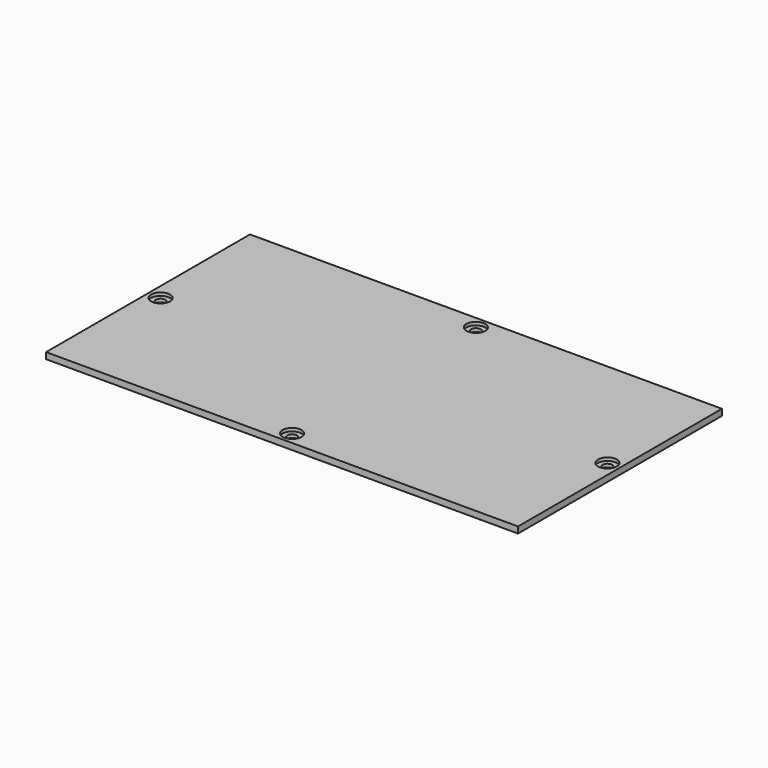
from build123d import *

# Parameters (mm, degrees)
F0_W     = 8
F0_H     = 8
F0_R     = 3
F1_DEPTH = 2
F0_R_2   = 1.5
F2_DEPTH = 1


# Not quite as in the source:
# - a feature names something its author has since deleted; it is built from what else it names


with BuildPart() as f1:
    # F0 (on Top) → F1 (new body)
    with BuildSketch(Plane.XY):
        Polygon((4, -40.5), (75, -40.5), (75, -4), (67, -4), (67, 4), (75, 4), (75, 40.5), (4, 40.5), (4, 32.5), (-4, 32.5), (-4, 40.5), (-75, 40.5), (-75, 4), (-67, 4), (-67, -4), (-75, -4), (-75, -40.5), (-4, -40.5), (-4, -32.5), (4, -32.5), align=None)
        with Locations((-71, 0)):
            Rectangle(F0_W, F0_H)
        with Locations((-71, 0)):
            Circle(F0_R, mode=Mode.SUBTRACT)
        with Locations((0, 36.5)):
            Rectangle(F0_W, F0_H)
        with Locations((0, 36.5)):
            Circle(F0_R, mode=Mode.SUBTRACT)
        with Locations((71, 0)):
            Rectangle(F0_W, F0_H)
        with Locations((71, 0)):
            Circle(F0_R, mode=Mode.SUBTRACT)
        with Locations((0, -36.5)):
            Rectangle(F0_W, F0_H)
        with Locations((0, -36.5)):
            Circle(F0_R, mode=Mode.SUBTRACT)
    extrude(amount=F1_DEPTH)

    # F0 (on Top) → F2 (join)
    with BuildSketch(Plane.XY):
        with Locations((0, 36.5)):
            Circle(F0_R)
        with Locations((0, 36.5)):
            Circle(F0_R_2, mode=Mode.SUBTRACT)
        with Locations((71, 0)):
            Circle(F0_R)
        with Locations((71, 0)):
            Circle(F0_R_2, mode=Mode.SUBTRACT)
        with Locations((0, -36.5)):
            Circle(F0_R)
        with Locations((0, -36.5)):
            Circle(F0_R_2, mode=Mode.SUBTRACT)
        with Locations((-71, 0)):
            Circle(F0_R)
        with Locations((-71, 0)):
            Circle(F0_R_2, mode=Mode.SUBTRACT)
    extrude(amount=F2_DEPTH)


solid = f1.part
